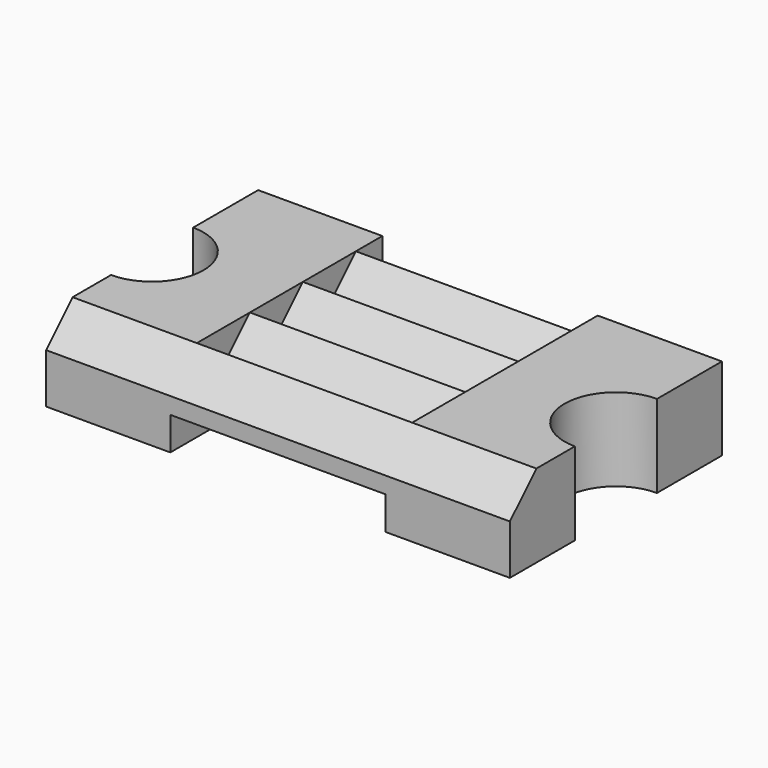
from build123d import *

# Parameters (mm, degrees)
F0_R     = 1.55
F1_DEPTH = 2.5
F3_DEPTH = 2.501
F4_W     = 6.5
F4_H     = 1
F5_DEPTH = 1
F6_W     = 6.5
F6_H     = 1
F7_DEPTH = 1
F8_SIZE  = 0.99999


# Not quite as in the source:
# - a fillet or chamfer is up to 0.001 mm smaller than in the source, because OpenCascade refuses the exact size


with BuildPart() as f1:
    # F0 (on Top) → F1 (new body)
    with BuildSketch(Plane.XY):
        with BuildLine():
            Line((7, 4), (-7, 4))
            ThreePointArc((-7, 4), (-9.8284271247, 2.8284271247), (-11, 0))
            ThreePointArc((-11, 0), (-9.8284271247, -2.8284271247), (-7, -4))
            Line((-7, -4), (7, -4))
            ThreePointArc((7, -4), (9.8284271247, -2.8284271247), (11, 0))
            ThreePointArc((11, 0), (9.8284271247, 2.8284271247), (7, 4))
        make_face()
        with Locations((-7, 0)):
            Circle(F0_R, mode=Mode.SUBTRACT)
        with Locations((7, 0)):
            Circle(F0_R, mode=Mode.SUBTRACT)
    extrude(amount=F1_DEPTH)

    # F2 (on face) → F3 (cut, through all)
    with BuildSketch(Plane.XY.offset(2.5)):
        with BuildLine():
            Line((-7, 1.55), (-7, 4))
            ThreePointArc((-7, 4), (-11, 0), (-7, -4))
            Line((-7, -4), (-7, -1.55))
            ThreePointArc((-7, -1.55), (-8.55, 0), (-7, 1.55))
        make_face()
        with BuildLine():
            ThreePointArc((7, -4), (11, 0), (7, 4))
            Line((7, 4), (7, 1.55))
            ThreePointArc((7, 1.55), (8.0960155108, 1.0960155108), (8.55, 0))
            ThreePointArc((8.55, 0), (8.0960155108, -1.0960155108), (7, -1.55))
            Line((7, -1.55), (7, -4))
        make_face()
    extrude(amount=-F3_DEPTH, mode=Mode.SUBTRACT)

    # F4 (on face) → F5 (cut)
    with BuildSketch(Plane.XY.offset(2.5)):
        with Locations((0, 1.5)):
            Rectangle(F4_W, F4_H)
        with Locations((0, -2.5)):
            Rectangle(F4_W, F4_H)
        with Locations((0, -0.5)):
            Rectangle(F4_W, F4_H)
        with Locations((0, 3.5)):
            Rectangle(F4_W, F4_H)
    extrude(amount=-F5_DEPTH, mode=Mode.SUBTRACT)

    # F6 (on face) → F7 (cut)
    with BuildSketch(Plane(origin=(0, 0, 0), x_dir=(1, 0, 0), z_dir=(0, 0, -1))):
        with Locations((0, -0.5)):
            Rectangle(F6_W, F6_H)
        with Locations((0, 3.5)):
            Rectangle(F6_W, F6_H)
        with Locations((0, 1.5)):
            Rectangle(F6_W, F6_H)
        with Locations((0, -2.5)):
            Rectangle(F6_W, F6_H)
    extrude(amount=-F7_DEPTH, mode=Mode.SUBTRACT)

    # F8 (size 1 in the source; OpenCascade refuses exactly that, so slightly less here)
    f8_edges = [f1.edges().sort_by_distance(p)[0] for p in [
        (0, 3, 0),
        (0, 1, 0),
        (0, -1, 0),
        (0, -3, 0),
        (0, -4, 2.5),
        (0, -2, 2.5),
        (0, 0, 2.5),
        (0, 2, 2.5),
    ]]
    chamfer(f8_edges, length=F8_SIZE)


solid = f1.part
